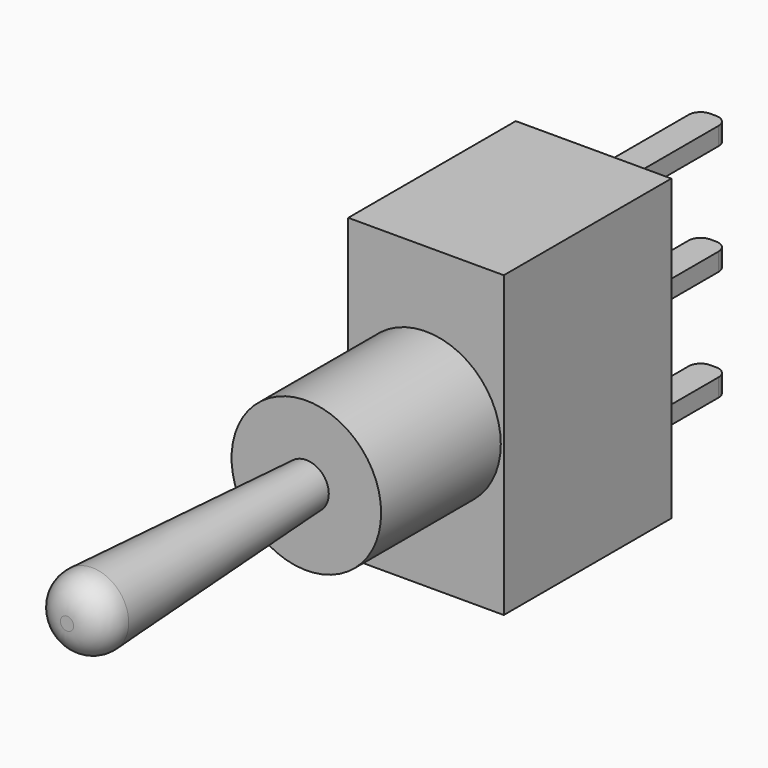
from build123d import *

# Parameters (mm, degrees)
F0_W     = 6.604
F0_H     = 12.7
F0_R     = 3.175
F1_DEPTH = 8.89
F2_DEPTH = 6.35
F3_R     = 0.9525
F4_DEPTH = 12.7
F4_TAPER = -3
F5_R     = 1.27
F6_W     = 1.27
F6_H     = 0.762
F7_DEPTH = 6.35
F8_R     = 0.508


with BuildPart() as f1:
    # F0 (on Front) → F1 (new body)
    with BuildSketch(Plane.XZ):
        Rectangle(F0_W, F0_H)
        Circle(F0_R, mode=Mode.SUBTRACT)
        Circle(F0_R)
    extrude(amount=-F1_DEPTH)

    # F0 (on Front) → F2 (join)
    with BuildSketch(Plane.XZ):
        Circle(F0_R)
    extrude(amount=F2_DEPTH)

    # F3 (on face) → F4 (join)
    with BuildSketch(Plane.XZ.offset(6.35)):
        Circle(F3_R)
    extrude(amount=F4_DEPTH, taper=F4_TAPER)

    # F5
    f5_edges = [f1.edges().sort_by_distance(p)[0] for p in [
        (-1.618079, -19.05, 0),
    ]]
    fillet(f5_edges, radius=F5_R)

    # F6 (on face) → F7 (join)
    with BuildSketch(Plane(origin=(0, 8.89, 0), x_dir=(-1, 0, 0), z_dir=(0, 1, 0))):
        with Locations((0, 4.699)):
            Rectangle(F6_W, F6_H)
        Rectangle(F6_W, F6_H)
        with Locations((0, -4.699)):
            Rectangle(F6_W, F6_H)
    extrude(amount=F7_DEPTH)

    # F8
    f8_edges = [f1.edges().sort_by_distance(p)[0] for p in [
        (0.635, 15.24, 4.699),
        (-0.635, 15.24, 4.699),
        (0.635, 15.24, 0),
        (-0.635, 15.24, 0),
        (0.635, 15.24, -4.699),
        (-0.635, 15.24, -4.699),
    ]]
    fillet(f8_edges, radius=F8_R)


solid = f1.part
